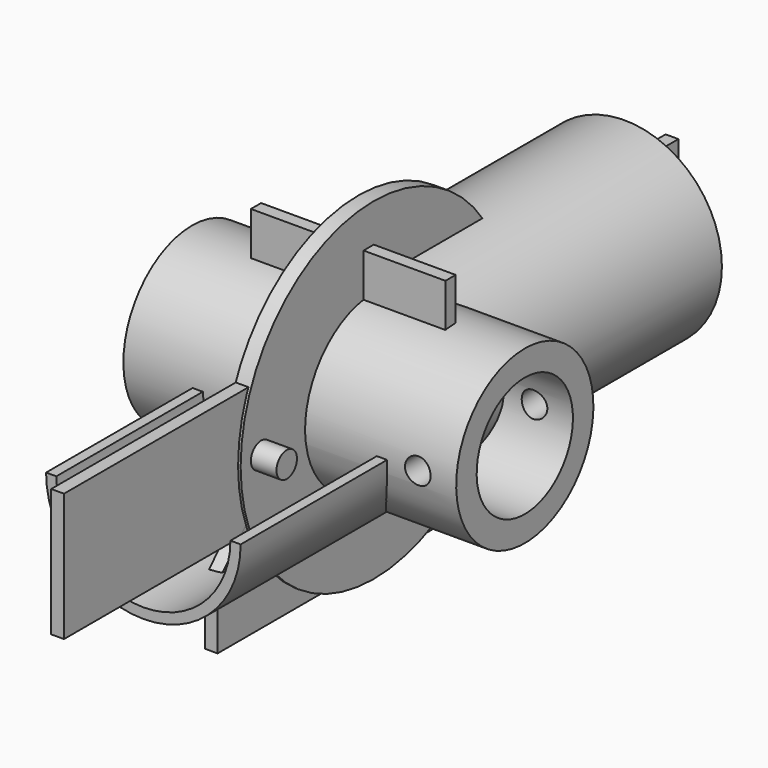
from build123d import *

# Parameters (mm, degrees)
F1_DEPTH  = 105
F2_DEPTH  = 130
F4_DEPTH  = 5
F5_W      = 65
F5_H      = 10
F7_DEPTH  = 34
F9_DEPTH  = 6
F10_DEPTH = 16
F11_R     = 5
F12_DEPTH = 33
F13_SIZE2 = 1
F13_SIZE  = 5
F14_SIZE2 = 5
F14_SIZE  = 1
F16_DEPTH = 3
F17_R     = 12.5
F18_DEPTH = 30
F19_W     = 300
F19_H     = 50
F20_DEPTH = 5
F22_DEPTH = 5


# Not quite as in the source:
# - a feature names something its author has since deleted; it is built from what else it names


with BuildPart() as f1:
    # F0 (on Front) → F1 (new body)
    with BuildSketch(Plane.XZ):
        with BuildLine():
            Line((38, 0), (34, 0))
            ThreePointArc((34, 0), (0, -34), (-34, 0))
            Line((-34, 0), (-38, 0))
            ThreePointArc((-38, 0), (0, -38), (38, 0))
        make_face()
    extrude(amount=F1_DEPTH)

    # F0 (on Front) → F2 (join)
    with BuildSketch(Plane.XZ):
        with BuildLine():
            Line((38, 0), (34, 0))
            ThreePointArc((34, 0), (0, -34), (-34, 0))
            Line((-34, 0), (-38, 0))
            ThreePointArc((-38, 0), (0, -38), (38, 0))
        make_face()
        with BuildLine():
            ThreePointArc((-34, 0), (0, 34), (34, 0))
            Line((34, 0), (38, 0))
            ThreePointArc((38, 0), (0, 38), (-38, 0))
            Line((-38, 0), (-34, 0))
        make_face()
    extrude(amount=-F2_DEPTH)


with BuildPart() as f4:
    # F3 (on Front) → F4 (new body)
    with BuildSketch(Plane.XZ):
        with BuildLine():
            ThreePointArc((-38, 0), (0, 38), (38, 0))
            Line((38, 0), (38, 50))
            Line((38, 50), (-38, 50))
            Line((-38, 50), (-38, 0))
        make_face()
        with BuildLine():
            ThreePointArc((-38, 0), (0, -38), (38, 0))
            Line((38, 0), (-38, 0))
        make_face()
        with BuildLine():
            Line((-38, 0), (38, 0))
            ThreePointArc((38, 0), (0, 38), (-38, 0))
        make_face()
    extrude(amount=F4_DEPTH)


with BuildPart() as f6:
    # F5 (on Front) → F6 (revolve)
    with BuildSketch(Plane.XZ):
        with Locations((32.5, 28.5)):
            Rectangle(F5_W, F5_H)
        Polygon((0, 23.5), (0, 33.5), (-65, 33.5), (-65, 0), (0, 0), align=None)
    revolve(axis=Axis((0, 0, 0), (1, 0, 0)))

    # F5 (on Front) → F7 (cut, symmetric)
    with BuildSketch(Plane.XZ):
        with BuildLine():
            ThreePointArc((45, 0), (50, -5), (55, 0))
            Line((55, 0), (45, 0))
        make_face()
        with BuildLine():
            Line((45, 0), (55, 0))
            ThreePointArc((55, 0), (50, 5), (45, 0))
        make_face()
    extrude(amount=F7_DEPTH, both=True, mode=Mode.SUBTRACT)


with BuildPart() as f9:
    # F8 (on Right) → F9 (new body)
    with BuildSketch(Plane.YZ):
        with BuildLine():
            Line((12.5, 0), (65, 0))
            ThreePointArc((65, 0), (0, 65), (-65, 0))
            Line((-65, 0), (-60, 0))
            ThreePointArc((-60, 0), (-55, 5), (-50, 0))
            Line((-50, 0), (-12.5, 0))
            ThreePointArc((-12.5, 0), (0, 12.5), (12.5, 0))
        make_face()
        with BuildLine():
            ThreePointArc((-65, 0), (0, -65), (65, 0))
            Line((65, 0), (12.5, 0))
            ThreePointArc((12.5, 0), (0, -12.5), (-12.5, 0))
            Line((-12.5, 0), (-50, 0))
            ThreePointArc((-50, 0), (-55, -5), (-60, 0))
            Line((-60, 0), (-65, 0))
        make_face()
    extrude(amount=F9_DEPTH)

    # F8 (on Right) → F10 (join)
    with BuildSketch(Plane.YZ):
        with BuildLine():
            Line((-50, 0), (-60, 0))
            ThreePointArc((-60, 0), (-55, -5), (-50, 0))
        make_face()
        with BuildLine():
            ThreePointArc((-50, 0), (-55, 5), (-60, 0))
            Line((-60, 0), (-50, 0))
        make_face()
    extrude(amount=F10_DEPTH)


with BuildPart() as f12:
    # F11 (on Right) → F12 (new body, symmetric)
    with BuildSketch(Plane.YZ):
        Circle(F11_R)
    extrude(amount=F12_DEPTH, both=True)

    # F13
    f13_edges = [f12.edges().sort_by_distance(p)[0] for p in [
        (33, -5, 0),
    ]]
    f13_side = f12.faces().sort_by_distance((33, 0, 0))[0]
    chamfer(f13_edges, length=F13_SIZE, length2=F13_SIZE2, reference=f13_side)

    # F14
    f14_edges = [f12.edges().sort_by_distance(p)[0] for p in [
        (-33, -5, 0),
    ]]
    chamfer(f14_edges, length=F14_SIZE, length2=F14_SIZE2)


with BuildPart() as f16:
    # F15 (on Right) → F16 (new body, symmetric)
    with BuildSketch(Plane.YZ):
        with BuildLine():
            Line((-85, 5), (-76.3397459622, 5))
            ThreePointArc((-76.3397459622, 5), (-95, 0), (-76.3397459622, -5))
            Line((-76.3397459622, -5), (-85, -5))
            ThreePointArc((-85, -5), (-90, 0), (-85, 5))
        make_face()
        with BuildLine():
            ThreePointArc((-75, 0), (-75.3407417371, 2.588190451), (-76.3397459622, 5))
            Line((-76.3397459622, 5), (-85, 5))
            ThreePointArc((-85, 5), (-81.4644660941, 3.5355339059), (-80, 0))
            ThreePointArc((-80, 0), (-81.4644660941, -3.5355339059), (-85, -5))
            Line((-85, -5), (-76.3397459622, -5))
            ThreePointArc((-76.3397459622, -5), (-75.3407417371, -2.588190451), (-75, 0))
        make_face()
        with BuildLine():
            ThreePointArc((76.3397459622, -5), (75, 0), (76.3397459622, 5))
            Line((76.3397459622, 5), (-76.3397459622, 5))
            ThreePointArc((-76.3397459622, 5), (-75.3407417371, 2.588190451), (-75, 0))
            ThreePointArc((-75, 0), (-75.3407417371, -2.588190451), (-76.3397459622, -5))
            Line((-76.3397459622, -5), (76.3397459622, -5))
        make_face()
        with BuildLine():
            ThreePointArc((85, -5), (80, 0), (85, 5))
            Line((85, 5), (76.3397459622, 5))
            ThreePointArc((76.3397459622, 5), (75, 0), (76.3397459622, -5))
            Line((76.3397459622, -5), (85, -5))
        make_face()
        with BuildLine():
            Line((76.3397459622, 5), (85, 5))
            ThreePointArc((85, 5), (88.5355339059, 3.5355339059), (90, 0))
            ThreePointArc((90, 0), (88.5355339059, -3.5355339059), (85, -5))
            Line((85, -5), (76.3397459622, -5))
            ThreePointArc((76.3397459622, -5), (87.588190451, -9.6592582629), (95, 0))
            ThreePointArc((95, 0), (87.588190451, 9.6592582629), (76.3397459622, 5))
        make_face()
    extrude(amount=F16_DEPTH, both=True)


with BuildPart() as f18:
    # F17 (on Right) → F18 (new body)
    with BuildSketch(Plane.YZ):
        Circle(F17_R)
    extrude(amount=F18_DEPTH)


with BuildPart() as f20:
    # F19 (on Right) → F20 (new body)
    with BuildSketch(Plane.YZ):
        Rectangle(F19_W, F19_H)
    extrude(amount=F20_DEPTH)


with BuildPart() as f22:
    # F21 (on Right) → F22 (new body)
    with BuildSketch(Plane.YZ):
        with BuildLine():
            Line((75, -36.1188948154), (40, 0))
            ThreePointArc((40, 0), (33.8195045896, -21.3598012471), (17.1879445342, -36.1188948154))
            Line((17.1879445342, -36.1188948154), (75, -36.1188948154))
        make_face()
        with BuildLine():
            Line((75, -36.1188948154), (17.1879445342, -36.1188948154))
            ThreePointArc((17.1879445342, -36.1188948154), (0, -40), (-17.1879445342, -36.1188948154))
            Line((-17.1879445342, -36.1188948154), (-75, -36.1188948154))
            Line((-75, -36.1188948154), (-75, -60.4170560837))
            Line((-75, -60.4170560837), (75, -60.4170560837))
            Line((75, -60.4170560837), (75, -36.1188948154))
        make_face()
        with BuildLine():
            ThreePointArc((-17.1879445342, -36.1188948154), (-33.8195045896, -21.3598012471), (-40, 0))
            Line((-40, 0), (-75, -36.1188948154))
            Line((-75, -36.1188948154), (-17.1879445342, -36.1188948154))
        make_face()
    extrude(amount=F22_DEPTH)


solid = Compound([f1.part, f4.part, f6.part, f9.part, f12.part, f16.part, f18.part, f20.part, f22.part])
